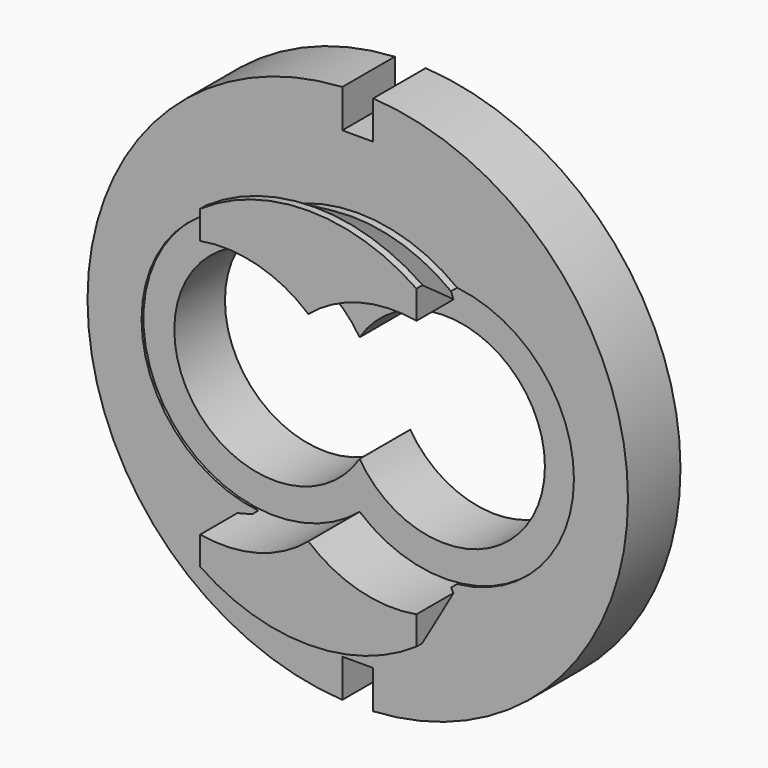
from build123d import *

# Parameters (mm, degrees)
F0_R      = 35
F1_DEPTH  = 8.5
F2_R      = 21.2425
F3_DEPTH  = 1
F4_R      = 21.2425
F5_DEPTH  = 6
F5_TAPER  = -30
F6_R      = 24.75
F7_DEPTH  = 1
F9_DEPTH  = 16.5
F11_DEPTH = 8.3
F12_W     = 12.0533492022
F12_H     = 52.1821774244
F12_W_2   = 10.4364354849
F12_H_2   = 52.770149804
F13_DEPTH = 8
F14_W     = 4
F14_H     = 6
F15_DEPTH = 8.5


# Not quite as in the source:
# - a pattern or mirror of a feature is missing from the dataset's text; its kind, count and spacing are read off the source's solid


with BuildPart() as f1:
    # F0 (on Front) → F1 (new body)
    with BuildSketch(Plane.XZ):
        Circle(F0_R)
    extrude(amount=F1_DEPTH)

    # F2 (on face) → F3 (join)
    with BuildSketch(Plane.XZ.offset(8.5)):
        Circle(F2_R)
    extrude(amount=F3_DEPTH)

    # F4 (on face) → F5 (join)
    with BuildSketch(Plane.XZ.offset(9.5)):
        Circle(F4_R)
    extrude(amount=F5_DEPTH, taper=F5_TAPER)

    # F6 (on face) → F7 (join)
    with BuildSketch(Plane.XZ.offset(15.5)):
        Circle(F6_R)
    extrude(amount=F7_DEPTH)

    # F8 (on face) → F9 (cut)
    with BuildSketch(Plane.XZ.offset(16.5)):
        with BuildLine():
            ThreePointArc((0, -6.9282032303), (1.4899959968, -3.6055512755), (2, 0))
            ThreePointArc((2, 0), (1.4899959968, 3.6055512755), (0, 6.9282032303))
            ThreePointArc((0, 6.9282032303), (-2, 0), (0, -6.9282032303))
        make_face()
        with BuildLine():
            ThreePointArc((0, 6.9282032303), (1.4899959968, 3.6055512755), (2, 0))
            ThreePointArc((2, 0), (1.4899959968, -3.6055512755), (0, -6.9282032303))
            ThreePointArc((0, -6.9282032303), (14.6055512755, -12.4899959968), (24, 0))
            ThreePointArc((24, 0), (14.6055512755, 12.4899959968), (0, 6.9282032303))
        make_face()
        with BuildLine():
            ThreePointArc((0, -6.9282032303), (-2, 0), (0, 6.9282032303))
            ThreePointArc((0, 6.9282032303), (-24, 0), (0, -6.9282032303))
        make_face()
    extrude(amount=-F9_DEPTH, mode=Mode.SUBTRACT)

    # F10 (on face) → F11 (cut)
    with BuildSketch(Plane.XZ.offset(16.5)):
        with BuildLine():
            ThreePointArc((0, -12.9614813968), (4.4272486205, -7.1414284285), (6, 0))
            ThreePointArc((6, 0), (4.4272486205, 7.1414284285), (0, 12.9614813968))
            ThreePointArc((0, 12.9614813968), (-6, 0), (0, -12.9614813968))
        make_face()
        with BuildLine():
            ThreePointArc((0, 12.9614813968), (4.4272486205, 7.1414284285), (6, 0))
            ThreePointArc((6, 0), (4.4272486205, -7.1414284285), (0, -12.9614813968))
            ThreePointArc((0, -12.9614813968), (18.1414284285, -15.4272486205), (28, 0))
            ThreePointArc((28, 0), (18.1414284285, 15.4272486205), (0, 12.9614813968))
        make_face()
        with BuildLine():
            ThreePointArc((0, -12.9614813968), (-6, 0), (0, 12.9614813968))
            ThreePointArc((0, 12.9614813968), (-28, 0), (0, -12.9614813968))
        make_face()
    extrude(amount=-F11_DEPTH, mode=Mode.SUBTRACT)

    # F12 (on face) → F13 (cut)
    with BuildSketch(Plane.XZ.offset(16.5)):
        with Locations((20.0266746011, 0.6560230852)):
            Rectangle(F12_W, F12_H)
        with Locations((-19.2182177424, 2.2729368025)):
            Rectangle(F12_W_2, F12_H_2)
    extrude(amount=-F13_DEPTH, mode=Mode.SUBTRACT)

    # F14 (on face) → F15 (cut)
    with BuildSketch(Plane.XZ.offset(8.5)):
        with Locations((0, 33)):
            Rectangle(F14_W, F14_H)
    f15 = extrude(amount=-F15_DEPTH, mode=Mode.SUBTRACT)

    # F15_copies: F15 across plane
    add(f15.mirror(Plane(origin=(0, 0, 0), x_dir=(-1, 0, 0), z_dir=(0, 0, -1))), mode=Mode.SUBTRACT)


solid = f1.part
